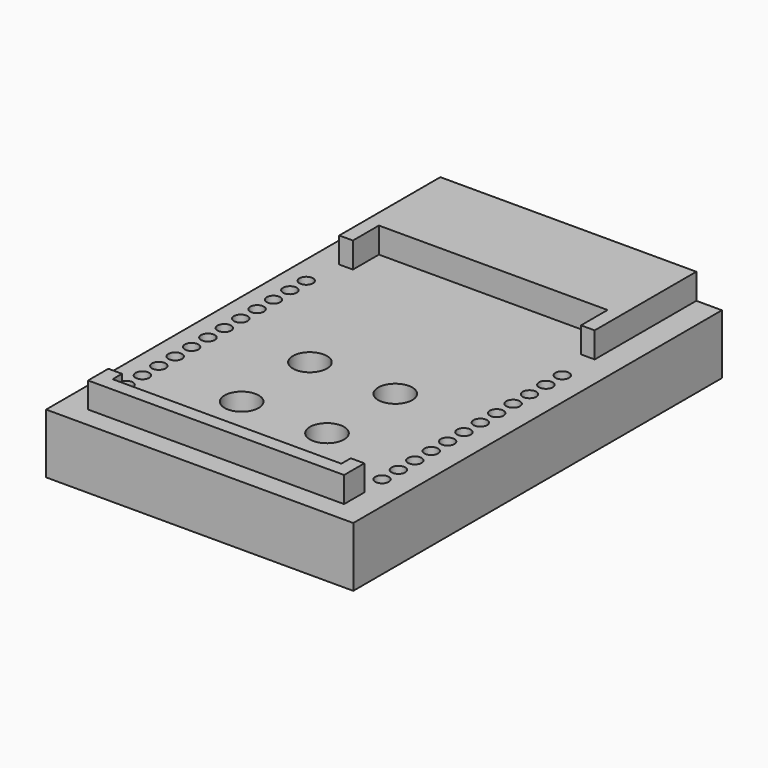
from build123d import *

# Parameters (mm, degrees)
F1_DEPTH = 5
F0_R     = 1
F2_DEPTH = 3.5
F3_R     = 0.4
F4_DEPTH = 12.5


with BuildPart() as f1:
    # F0 (on Top) → F1 (new body)
    with BuildSketch(Plane.XY):
        Polygon((0, 1.4873089967), (0, 0), (15, 0), (15, 1.4873089967), (14.2, 1.4873089967), (14.2, 0.8), (0.8, 0.8), (0.8, 1.4873089967), align=None)
    extrude(amount=F1_DEPTH)

    # F0 (on Top) → F2 (join)
    with BuildSketch(Plane.XY):
        Polygon((0, 18.3973629028), (0, 25.8), (-1.5, 25.8), (-1.5, -1.2), (16.5, -1.2), (16.5, 25.8), (15, 25.8), (15, 18.3544885367), (14.2, 18.3544885367), (14.2, 20.3), (0.8, 20.3), (0.8, 18.3973629028), align=None)
        with Locations((5, 5)):
            Circle(F0_R, mode=Mode.SUBTRACT)
        with Locations((5, 10)):
            Circle(F0_R, mode=Mode.SUBTRACT)
        Polygon((15, 0), (0, 0), (0, 1.4873089967), (0.8, 1.4873089967), (0.8, 0.8), (14.2, 0.8), (14.2, 1.4873089967), (15, 1.4873089967), align=None, mode=Mode.SUBTRACT)
        with Locations((10, 5)):
            Circle(F0_R, mode=Mode.SUBTRACT)
        with Locations((10, 10)):
            Circle(F0_R, mode=Mode.SUBTRACT)
    extrude(amount=F2_DEPTH)

    # F3 (on face) → F4 (cut, symmetric)
    with BuildSketch(Plane.XY.offset(3.5)):
        with Locations((-0.175, 3)):
            Circle(F3_R)
        with Locations((-0.175, 4.2)):
            Circle(F3_R)
        with Locations((-0.175, 5.4)):
            Circle(F3_R)
        with Locations((-0.175, 6.6)):
            Circle(F3_R)
        with Locations((-0.175, 7.8)):
            Circle(F3_R)
        with Locations((-0.175, 9)):
            Circle(F3_R)
        with Locations((-0.175, 10.2)):
            Circle(F3_R)
        with Locations((-0.175, 11.4)):
            Circle(F3_R)
        with Locations((-0.175, 12.6)):
            Circle(F3_R)
        with Locations((-0.175, 13.8)):
            Circle(F3_R)
        with Locations((-0.175, 15)):
            Circle(F3_R)
        with Locations((-0.175, 16.2)):
            Circle(F3_R)
        with Locations((14.825, 3)):
            Circle(F3_R)
        with Locations((14.825, 4.2)):
            Circle(F3_R)
        with Locations((14.825, 5.4)):
            Circle(F3_R)
        with Locations((14.825, 6.6)):
            Circle(F3_R)
        with Locations((14.825, 7.8)):
            Circle(F3_R)
        with Locations((14.825, 9)):
            Circle(F3_R)
        with Locations((14.825, 10.2)):
            Circle(F3_R)
        with Locations((14.825, 11.4)):
            Circle(F3_R)
        with Locations((14.825, 12.6)):
            Circle(F3_R)
        with Locations((14.825, 13.8)):
            Circle(F3_R)
        with Locations((14.825, 15)):
            Circle(F3_R)
        with Locations((14.825, 16.2)):
            Circle(F3_R)
    extrude(amount=F4_DEPTH, both=True, mode=Mode.SUBTRACT)


with BuildPart() as f1b:
    # F0 (on Top) → F1, piece 2 (new body)
    with BuildSketch(Plane.XY):
        Polygon((15, 25.8), (0, 25.8), (0, 18.3973629028), (0.8, 18.3973629028), (0.8, 20.3), (14.2, 20.3), (14.2, 18.3544885367), (15, 18.3544885367), align=None)
    extrude(amount=F1_DEPTH)


solid = Compound([f1.part, f1b.part])
